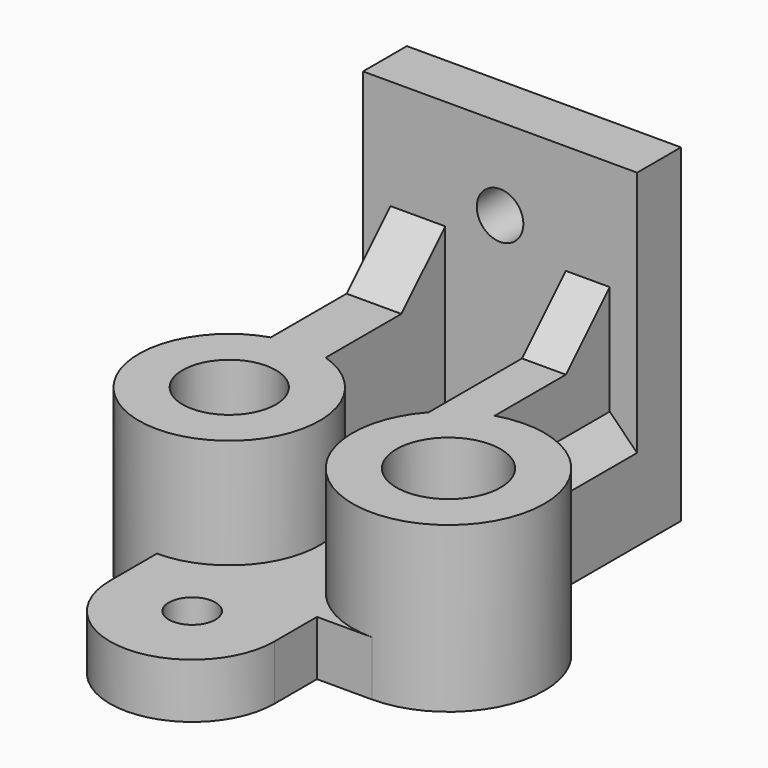
from build123d import *

# Parameters (mm, degrees)
F0_R          = 2.125
F0_R_2        = 4.25
F0_R_3        = 4.75
F1_DEPTH      = 5
F2_W          = 25
F2_H          = 5
F3_DEPTH      = 25
F4_R          = 8.25
F4_R_2        = 4.25
F4_R_3        = 8.75
F4_R_4        = 4.75
F5_DEPTH      = 10
F6_R          = 2.125
F7_DEPTH      = 5.001
F8_W          = 5
F8_H          = 13.6379074032
F8_W_2        = 4
F8_H_2        = 15.6423127431
F9_DEPTH      = 10
F10_T1_DEPTH  = 5
F10_T3_DEPTH  = 4
F10_T8_DEPTH  = 17.8584149398
F10_T13_DEPTH = 16.8584149398
F10_T18_DEPTH = 26.4963223431
F10_S19_R     = 8.25
F10_T20_DEPTH = 15
F10_T25_DEPTH = 26.4963223431
F10_S26_R     = 8.25
F10_T27_DEPTH = 15
F10_T32_DEPTH = 25.9731600242
F10_S34_R     = 8.75
F10_T35_DEPTH = 15


# Not quite as in the source:
# - a fillet or chamfer that OpenCascade refuses, or shapes differently, is made with other operations: its cross-section is extruded or revolved along the edge and cut away or added


with BuildPart() as f1:
    # F0 (on Top) → F1 (new body)
    with BuildSketch(Plane.XY):
        with BuildLine():
            Line((12.5, 26.5), (0, 26.5))
            Line((0, 26.5), (-12.5, 26.5))
            Line((-12.5, 26.5), (-12.5, 6.5622023742))
            ThreePointArc((-12.5, 6.5622023742), (-15.3166703137, -2.6385915194), (-7.5, -8.25))
            Line((-7.5, -8.25), (-7.5, -13.6))
            ThreePointArc((-7.5, -13.6), (-5.3033008589, -18.9033008589), (0, -21.1))
            ThreePointArc((0, -21.1), (5.3033008589, -18.9033008589), (7.5, -13.6))
            Line((7.5, -13.6), (7.5, -8.75))
            Line((7.5, -8.75), (12.5, -8.75))
            ThreePointArc((12.5, -8.75), (21.25, 0), (12.5, 8.75))
            Line((12.5, 8.75), (12.5, 26.5))
        make_face()
        with Locations((0, -13.6)):
            Circle(F0_R, mode=Mode.SUBTRACT)
        with Locations((-7.5, 0)):
            Circle(F0_R_2, mode=Mode.SUBTRACT)
        with Locations((12.5, 0)):
            Circle(F0_R_3, mode=Mode.SUBTRACT)
        with Locations((0, 16.5)):
            Circle(F0_R, mode=Mode.SUBTRACT)
    extrude(amount=F1_DEPTH)

    # F2 (on face) → F3 (join)
    with BuildSketch(Plane.XY.offset(5)):
        with Locations((0, 24)):
            Rectangle(F2_W, F2_H)
    extrude(amount=F3_DEPTH)

    # F4 (on face) → F5 (join)
    with BuildSketch(Plane.XY.offset(5)):
        with Locations((-7.5, 0)):
            Circle(F4_R)
        with Locations((-7.5, 0)):
            Circle(F4_R_2, mode=Mode.SUBTRACT)
        with Locations((12.5, 0)):
            Circle(F4_R_3)
        with Locations((12.5, 0)):
            Circle(F4_R_4, mode=Mode.SUBTRACT)
    extrude(amount=F5_DEPTH)

    # F6 (on face) → F7 (cut, through all)
    with BuildSketch(Plane.XZ.offset(-21.5)):
        with Locations((0, 22.5)):
            Circle(F6_R)
    extrude(amount=-F7_DEPTH, mode=Mode.SUBTRACT)

    # F8 (on face) → F9 (join)
    with BuildSketch(Plane.XY.offset(5)):
        with Locations((-7.5, 14.6810462984)):
            Rectangle(F8_W, F8_H)
        with Locations((8, 13.6788436285)):
            Rectangle(F8_W_2, F8_H_2)
    extrude(amount=F9_DEPTH)

    # F10: chamfer of 5 on 4 edges, made by hand

    # F10_s2 → F10_t1 (join)
    with BuildSketch(Plane.YZ.offset(-10)):
        Polygon((21.5, 20), (16.5, 15), (21.5, 15), align=None)
    extrude(amount=F10_T1_DEPTH)

    # F10_s4 → F10_t3 (join)
    with BuildSketch(Plane.YZ.offset(6)):
        Polygon((21.5, 20), (16.5, 15), (21.5, 15), align=None)
    extrude(amount=F10_T3_DEPTH)


with BuildPart() as f10_tool6:
    # F10_s7 → F10_t8 (new body)
    with BuildSketch(Plane.YZ.offset(7.8584149398)):
        Polygon((21.5, 20), (16.5, 15), (21.5, 15), align=None)
    extrude(amount=-F10_T8_DEPTH)

    split(bisect_by=Plane.YZ.offset(6), keep=Keep.TOP)


with BuildPart() as f1_1:
    add(f1.part)

    # F10_t5: union F10_tool6
    add(f10_tool6.part)


with BuildPart() as f10_tool11:
    # F10_s12 → F10_t13 (new body)
    with BuildSketch(Plane.YZ.offset(10)):
        Polygon((21.5, 20), (16.5, 15), (21.5, 15), align=None)
    extrude(amount=-F10_T13_DEPTH)

    split(bisect_by=Plane.YZ.offset(-5), keep=Keep.BOTTOM)


with BuildPart() as f1_2:
    add(f1_1.part)

    # F10_t10: union F10_tool11
    add(f10_tool11.part)


with BuildPart() as f10_tool16:
    # F10_s17 → F10_t18 (new body)
    with BuildSketch(Plane.XZ.offset(-21.5)):
        Polygon((-10, 10), (-15, 5), (-10, 5), align=None)
    extrude(amount=F10_T18_DEPTH)

    # F10_s19 → F10_t20 (cut, symmetric)
    with BuildSketch(Plane.XY.offset(7.5)):
        with Locations((-7.5, 0)):
            Circle(F10_S19_R)
    extrude(amount=F10_T20_DEPTH, both=True, mode=Mode.SUBTRACT)

    split(bisect_by=Plane.YZ.offset(-12.5), keep=Keep.TOP)


with BuildPart() as f1_3:
    add(f1_2.part)

    # F10_t15: union F10_tool16
    add(f10_tool16.part)


with BuildPart() as f10_tool23:
    # F10_s24 → F10_t25 (new body)
    with BuildSketch(Plane.XZ.offset(-21.5)):
        Polygon((-10, 10), (-15, 5), (-10, 5), align=None)
    extrude(amount=F10_T25_DEPTH)

    # F10_s26 → F10_t27 (intersect, symmetric)
    with BuildSketch(Plane.XY.offset(7.5)):
        with Locations((-7.5, 0)):
            Circle(F10_S26_R)
    extrude(amount=F10_T27_DEPTH, both=True, mode=Mode.INTERSECT)

    split(bisect_by=Plane.YZ.offset(-12.5), keep=Keep.BOTTOM)


with BuildPart() as f1_4:
    add(f1_3.part)

    # F10_t22: union F10_tool23
    add(f10_tool23.part)


with BuildPart() as f10_tool30:
    # F10_s31 → F10_t32 (new body)
    with BuildSketch(Plane.XZ.offset(4.4731600242)):
        Polygon((15, 5), (10, 10), (10, 5), align=None)
    extrude(amount=-F10_T32_DEPTH)

    split(bisect_by=Plane.YZ.offset(12.5), keep=Keep.BOTTOM)

    # F10_s34 → F10_t35 (cut, symmetric)
    with BuildSketch(Plane.XY.offset(7.5)):
        with Locations((12.5, 0)):
            Circle(F10_S34_R)
    extrude(amount=F10_T35_DEPTH, both=True, mode=Mode.SUBTRACT)


with BuildPart() as f1_5:
    add(f1_4.part)

    # F10_t29: union F10_tool30
    add(f10_tool30.part)


solid = f1_5.part
